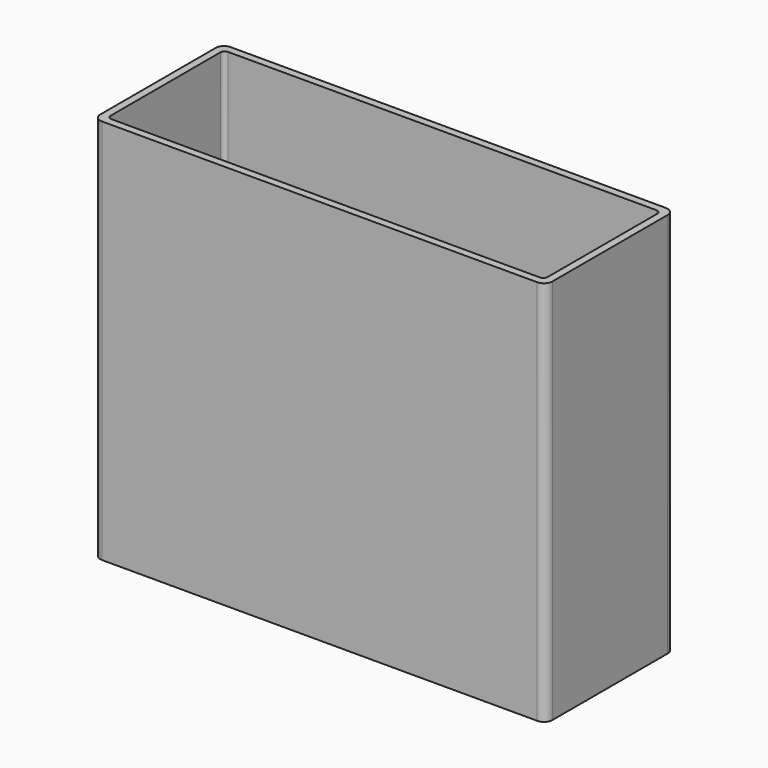
from build123d import *

# Parameters (mm, degrees)
F1_DEPTH = 91.44
F3_DEPTH = 38.608
F5_DEPTH = 4.7752
F6_R     = 1.35255
F7_DEPTH = 52.832


# Not quite as in the source:
# - a feature names something its author has since deleted; it is built from what else it names


with BuildPart() as f1:
    # F0 (on Top) → F1 (new body)
    with BuildSketch(Plane.XY):
        with BuildLine():
            ThreePointArc((0, 2), (0.5857864376, 0.5857864376), (2, 0))
            Line((2, 0), (105.061, 0))
            ThreePointArc((105.061, 0), (106.4752135624, 0.5857864376), (107.061, 2))
            Line((107.061, 2), (107.061, 36.1))
            ThreePointArc((107.061, 36.1), (106.4752135624, 37.5142135624), (105.061, 38.1))
            Line((105.061, 38.1), (2, 38.1))
            ThreePointArc((2, 38.1), (0.5857864376, 37.5142135624), (0, 36.1))
            Line((0, 36.1), (0, 2))
        make_face()
    extrude(amount=F1_DEPTH)

    # F2 (on face) → F3 (cut)
    with BuildSketch(Plane.XY.offset(91.44)):
        with BuildLine():
            Line((104.261, 36.3), (2.8, 36.3))
            ThreePointArc((2.8, 36.3), (2.0928932188, 36.0071067812), (1.8, 35.3))
            Line((1.8, 35.3), (1.8, 2.8))
            ThreePointArc((1.8, 2.8), (2.0928932188, 2.0928932188), (2.8, 1.8))
            Line((2.8, 1.8), (104.261, 1.8))
            ThreePointArc((104.261, 1.8), (104.9681067812, 2.0928932188), (105.261, 2.8))
            Line((105.261, 2.8), (105.261, 35.3))
            ThreePointArc((105.261, 35.3), (104.9681067812, 36.0071067812), (104.261, 36.3))
        make_face()
    extrude(amount=-F3_DEPTH, mode=Mode.SUBTRACT)

    # F4 (on face) → F5 (join)
    with BuildSketch(Plane(origin=(0, 0, 0), x_dir=(1, 0, 0), z_dir=(0, 0, -1))):
        with BuildLine():
            ThreePointArc((107.061, -2), (106.4752135624, -0.5857864376), (105.061, 0))
            Line((105.061, 0), (101.251, 0))
            Line((101.251, 0), (101.251, -2))
            ThreePointArc((101.251, -2), (102.3669231637, -4.6940768363), (105.061, -5.81))
            Line((105.061, -5.81), (107.061, -5.81))
            Line((107.061, -5.81), (107.061, -2))
        make_face()
        with BuildLine():
            Line((101.251, -36.1), (101.251, -38.1))
            Line((101.251, -38.1), (105.061, -38.1))
            ThreePointArc((105.061, -38.1), (106.4752135624, -37.5142135624), (107.061, -36.1))
            Line((107.061, -36.1), (107.061, -32.29))
            Line((107.061, -32.29), (105.061, -32.29))
            ThreePointArc((105.061, -32.29), (102.3669231637, -33.4059231637), (101.251, -36.1))
        make_face()
        with BuildLine():
            ThreePointArc((5.81, -36.1), (4.6940768363, -33.4059231637), (2, -32.29))
            Line((2, -32.29), (0, -32.29))
            Line((0, -32.29), (0, -36.1))
            ThreePointArc((0, -36.1), (0.5857864376, -37.5142135624), (2, -38.1))
            Line((2, -38.1), (5.81, -38.1))
            Line((5.81, -38.1), (5.81, -36.1))
        make_face()
        with BuildLine():
            Line((5.81, 0), (2, 0))
            ThreePointArc((2, 0), (0.5857864376, -0.5857864376), (0, -2))
            Line((0, -2), (0, -5.81))
            Line((0, -5.81), (2, -5.81))
            ThreePointArc((2, -5.81), (4.6940768363, -4.6940768363), (5.81, -2))
            Line((5.81, -2), (5.81, 0))
        make_face()
    extrude(amount=-F5_DEPTH)

    # F6 (on face) → F7 (cut, through all)
    with BuildSketch(Plane(origin=(0, 0, 0), x_dir=(1, 0, 0), z_dir=(0, 0, -1))):
        with Locations((103.8037641431, -3.2572358569)):
            Circle(F6_R)
        with Locations((3.2572358569, -3.2572358569)):
            Circle(F6_R)
        with Locations((3.2572358569, -34.8427641431)):
            Circle(F6_R)
        with Locations((103.8037641431, -34.8427641431)):
            Circle(F6_R)
    extrude(amount=-F7_DEPTH, mode=Mode.SUBTRACT)


solid = f1.part
